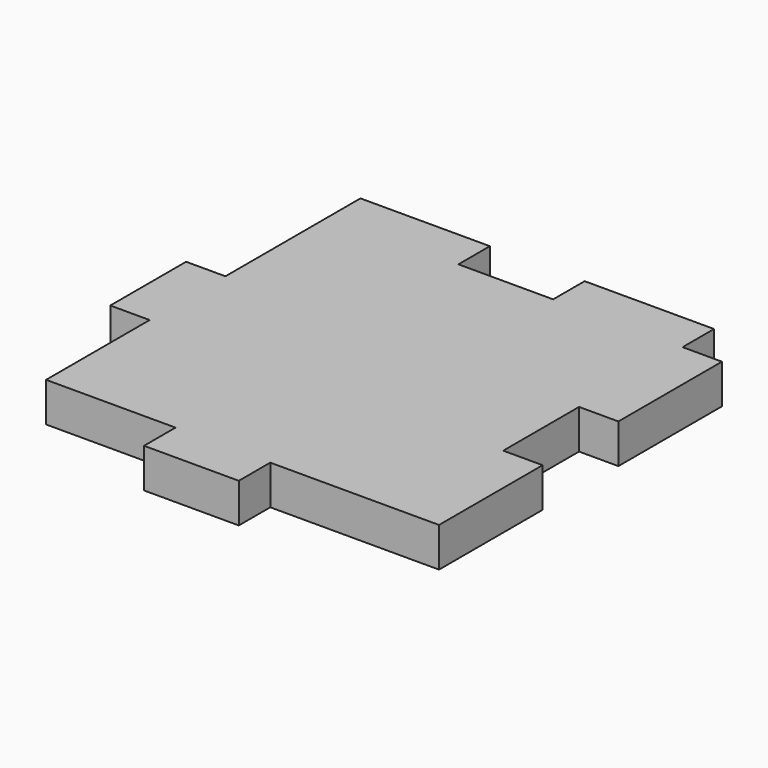
from build123d import *

# Parameters (mm, degrees)
F1_DEPTH = 4.45


# Not quite as in the source:
# - ends of sketch curves that miss each other by under 0.0002 mm in the source are joined


with BuildPart() as f1:
    # F0 (on Top) → F1 (new body)
    with BuildSketch(Plane.XY):
        Polygon((5.359896815, -20), (20, -20), (24.450000447, -20), (24.450000447, -5.3598965915), (20.000000447, -5.3598965915), (20.000000447, 5.3598965915), (24.450000447, 5.3598965915), (24.450000447, 20), (20, 20), (20.000000447, 24.45), (5.359896815, 24.45), (5.359896815, 20), (-5.359896368, 20), (-5.359896368, 24.45), (-20, 24.45), (-20, 20), (-20, 5.3598965915), (-24.450000447, 5.3598965915), (-24.450000447, -5.3598965915), (-20, -5.3598965915), (-20, -20), (-5.359896368, -20), (-5.359896368, -24.45), (5.359896815, -24.45), align=None)
    extrude(amount=F1_DEPTH)


solid = f1.part
